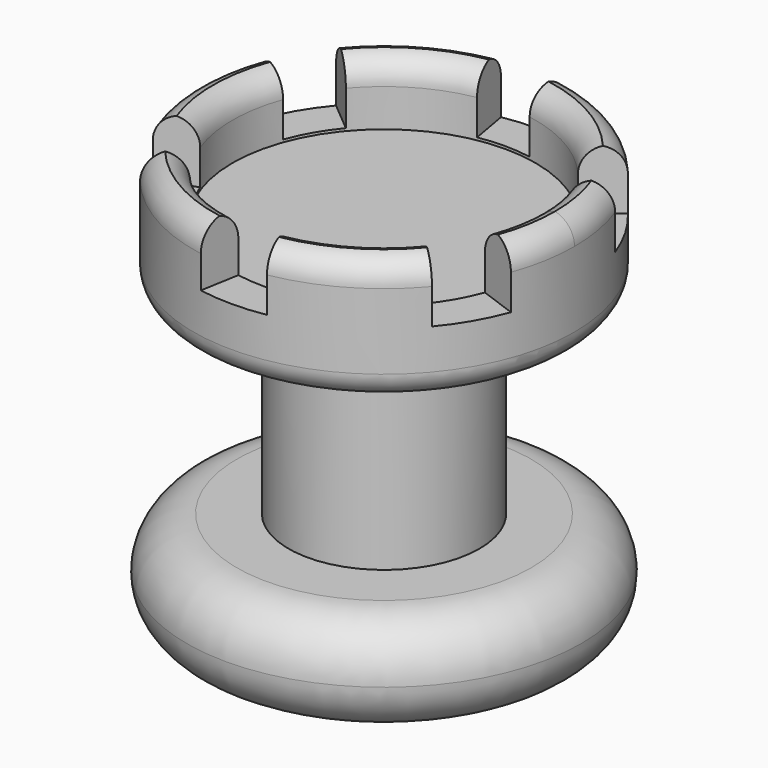
from build123d import *

# Parameters (mm, degrees)
F2_R          = 30.151436764
F3_DEPTH      = 12.5
F5_DEPTH      = 12
F6_R          = 9.99999
F7_T2_ANGLE   = 40
F7_T4_ANGLE   = 40
F8_T2_ANGLE   = 56.7791956191
F8_T4_ANGLE   = 61.1048655433
F9_T2_ANGLE   = 40
F9_T4_ANGLE   = 40
F10_T3_ANGLE  = 20
F10_T6_ANGLE  = 20
F10_T9_ANGLE  = 20
F10_T12_ANGLE = 20
F11_T2_ANGLE  = 40
F11_T4_ANGLE  = 40
F12_T2_ANGLE  = 87.5104431526
F12_T4_ANGLE  = 77.7726651693
F13_R         = 5


# Not quite as in the source:
# - a fillet or chamfer that OpenCascade refuses, or shapes differently, is made with other operations: its cross-section is extruded or revolved along the edge and cut away or added
# - a fillet or chamfer is up to 0.001 mm smaller than in the source, because OpenCascade refuses the exact size


with BuildPart() as f1:
    # F0 (on Front) → F1 (revolve)
    with BuildSketch(Plane.XZ):
        Polygon((0, 20), (0, 0), (19, 0), (39.2987092885, 0), (39.2987092885, 20), (19, 20), (19, 59.1294809732), (37.9244651105, 59.1294809732), (37.9244651105, 84.1294809732), (0, 84.1294809732), (0, 59.1294809732), align=None)
    revolve(axis=Axis((0, 0, 29.5647404866), (0, 0, 1)))

    # F2 (on face) → F3 (cut, symmetric)
    with BuildSketch(Plane.XY.offset(84.1294809732)):
        Circle(F2_R)
    extrude(amount=F3_DEPTH, both=True, mode=Mode.SUBTRACT)

    # F4 (on face) → F5 (cut)
    with BuildSketch(Plane.XY.offset(84.1294809732)):
        with BuildLine():
            ThreePointArc((-4.2811336318, 24.2795153332), (0, 24.654065993), (4.2811336318, 24.2795153332))
            Line((4.2811336318, 24.2795153332), (8.0445966017, 45.6231744531))
            ThreePointArc((8.0445966017, 45.6231744531), (0, 46.3269854584), (-8.0445966017, 45.6231744531))
            Line((-8.0445966017, 45.6231744531), (-4.2811336318, 24.2795153332))
        make_face()
        with BuildLine():
            ThreePointArc((-23.167243886, 8.4321871845), (-21.3510474565, 12.3270329965), (-18.8861102542, 15.8473281487))
            Line((-18.8861102542, 15.8473281487), (-35.4885297769, 29.7784122468))
            ThreePointArc((-35.4885297769, 29.7784122468), (-40.1203462877, 23.1634927292), (-43.5331263785, 15.8447622063))
            Line((-43.5331263785, 15.8447622063), (-23.167243886, 8.4321871845))
        make_face()
        with BuildLine():
            ThreePointArc((-18.8861102542, -15.8473281487), (-21.3510474565, -12.3270329965), (-23.167243886, -8.4321871845))
            Line((-23.167243886, -8.4321871845), (-43.5331263785, -15.8447622063))
            ThreePointArc((-43.5331263785, -15.8447622063), (-40.1203462877, -23.1634927292), (-35.4885297769, -29.7784122468))
            Line((-35.4885297769, -29.7784122468), (-18.8861102542, -15.8473281487))
        make_face()
        with BuildLine():
            ThreePointArc((4.2811336318, -24.2795153332), (0, -24.654065993), (-4.2811336318, -24.2795153332))
            Line((-4.2811336318, -24.2795153332), (-8.0445966017, -45.6231744531))
            ThreePointArc((-8.0445966017, -45.6231744531), (0, -46.3269854584), (8.0445966017, -45.6231744531))
            Line((8.0445966017, -45.6231744531), (4.2811336318, -24.2795153332))
        make_face()
        with BuildLine():
            ThreePointArc((23.167243886, -8.4321871845), (21.3510474565, -12.3270329965), (18.8861102542, -15.8473281487))
            Line((18.8861102542, -15.8473281487), (35.4885297769, -29.7784122468))
            ThreePointArc((35.4885297769, -29.7784122468), (40.1203462877, -23.1634927292), (43.5331263785, -15.8447622063))
            Line((43.5331263785, -15.8447622063), (23.167243886, -8.4321871845))
        make_face()
        with BuildLine():
            ThreePointArc((18.8861102542, 15.8473281487), (21.3510474565, 12.3270329965), (23.167243886, 8.4321871845))
            Line((23.167243886, 8.4321871845), (43.5331263785, 15.8447622063))
            ThreePointArc((43.5331263785, 15.8447622063), (40.1203462877, 23.1634927292), (35.4885297769, 29.7784122468))
            Line((35.4885297769, 29.7784122468), (18.8861102542, 15.8473281487))
        make_face()
    extrude(amount=-F5_DEPTH, mode=Mode.SUBTRACT)

    # F6 (radius 10 in the source; OpenCascade refuses exactly that, so slightly less here)
    f6_edges = [f1.edges().sort_by_distance(p)[0] for p in [
        (-39.298709, 0, 20),
        (-39.298709, 0, 0),
    ]]
    fillet(f6_edges, radius=F6_R)

    # F7: fillet of radius 5 on 2 edges, made by hand

    # F7_s1 → F7_t2 (revolve, cut)
    with BuildSketch(Plane(origin=(0, 0, 0), x_dir=(0, 0, 1), z_dir=(-0.984807753, -0.1736481777, 0))):
        with BuildLine():
            ThreePointArc((79.1294809732, -37.9244651105), (82.6650148792, -36.4599990164), (84.1294809732, -32.9244651105))
            Line((84.1294809732, -32.9244651105), (84.2294809732, -32.9244651105))
            Line((84.2294809732, -32.9244651105), (84.2294809732, -38.0244651105))
            Line((84.2294809732, -38.0244651105), (79.1294809732, -38.0244651105))
            Line((79.1294809732, -38.0244651105), (79.1294809732, -37.9244651105))
        make_face()
    revolve(axis=Axis((0, 0, 84.1294809732), (0, 0, 1)), revolution_arc=F7_T2_ANGLE, mode=Mode.SUBTRACT)

    # F7_s3 → F7_t4 (revolve, cut)
    with BuildSketch(Plane(origin=(0, 0, 0), x_dir=(0, 0, 1), z_dir=(-0.984807753, -0.1736481777, 0))):
        with BuildLine():
            ThreePointArc((84.1294809732, -35.151436764), (82.6650148792, -31.615902858), (79.1294809732, -30.151436764))
            Line((79.1294809732, -30.151436764), (79.1294809732, -30.051436764))
            Line((79.1294809732, -30.051436764), (84.2294809732, -30.051436764))
            Line((84.2294809732, -30.051436764), (84.2294809732, -35.151436764))
            Line((84.2294809732, -35.151436764), (84.1294809732, -35.151436764))
        make_face()
    revolve(axis=Axis((0, 0, 84.1294809732), (0, 0, 1)), revolution_arc=F7_T4_ANGLE, mode=Mode.SUBTRACT)

    # F8: fillet of radius 5.5526911935 on 2 edges, made by hand

    # F8_s1 → F8_t2 (revolve, cut)
    with BuildSketch(Plane(origin=(0, 0, 0), x_dir=(0, 0, 1), z_dir=(-0.5241405305, 0.8516317892, 0))):
        with BuildLine():
            ThreePointArc((78.5767897798, -37.9244651105), (82.5031353765, -36.2981195138), (84.1294809732, -32.371773917))
            Line((84.1294809732, -32.371773917), (84.2405347971, -32.371773917))
            Line((84.2405347971, -32.371773917), (84.2405347971, -38.0355189344))
            Line((84.2405347971, -38.0355189344), (78.5767897798, -38.0355189344))
            Line((78.5767897798, -38.0355189344), (78.5767897798, -37.9244651105))
        make_face()
    revolve(axis=Axis((0, 0, 84.1294809732), (0, 0, 1)), revolution_arc=F8_T2_ANGLE, mode=Mode.SUBTRACT)

    # F8_s3 → F8_t4 (revolve, cut)
    with BuildSketch(Plane(origin=(0, 0, 0), x_dir=(0, 0, 1), z_dir=(-0.4916268702, 0.8708059603, 0))):
        with BuildLine():
            ThreePointArc((84.1294809732, -35.7041279574), (82.5031353765, -31.7777823607), (78.5767897798, -30.151436764))
            Line((78.5767897798, -30.151436764), (78.5767897798, -30.0403829401))
            Line((78.5767897798, -30.0403829401), (84.2405347971, -30.0403829401))
            Line((84.2405347971, -30.0403829401), (84.2405347971, -35.7041279574))
            Line((84.2405347971, -35.7041279574), (84.1294809732, -35.7041279574))
        make_face()
    revolve(axis=Axis((0, 0, 84.1294809732), (0, 0, 1)), revolution_arc=F8_T4_ANGLE, mode=Mode.SUBTRACT)

    # F9: fillet of radius 5 on 2 edges, made by hand

    # F9_s1 → F9_t2 (revolve, cut)
    with BuildSketch(Plane(origin=(0, 0, 0), x_dir=(0, 0, 1), z_dir=(0.3420201433, 0.9396926208, 0))):
        with BuildLine():
            ThreePointArc((84.1294809732, -35.151436764), (82.6650148792, -31.615902858), (79.1294809732, -30.151436764))
            Line((79.1294809732, -30.151436764), (79.1294809732, -30.051436764))
            Line((79.1294809732, -30.051436764), (84.2294809732, -30.051436764))
            Line((84.2294809732, -30.051436764), (84.2294809732, -35.151436764))
            Line((84.2294809732, -35.151436764), (84.1294809732, -35.151436764))
        make_face()
    revolve(axis=Axis((0, 0, 84.1294809732), (0, 0, 1)), revolution_arc=F9_T2_ANGLE, mode=Mode.SUBTRACT)

    # F9_s3 → F9_t4 (revolve, cut)
    with BuildSketch(Plane(origin=(0, 0, 0), x_dir=(0, 0, 1), z_dir=(0.3420201433, 0.9396926208, 0))):
        with BuildLine():
            ThreePointArc((79.1294809732, -37.9244651105), (82.6650148792, -36.4599990164), (84.1294809732, -32.9244651105))
            Line((84.1294809732, -32.9244651105), (84.2294809732, -32.9244651105))
            Line((84.2294809732, -32.9244651105), (84.2294809732, -38.0244651105))
            Line((84.2294809732, -38.0244651105), (79.1294809732, -38.0244651105))
            Line((79.1294809732, -38.0244651105), (79.1294809732, -37.9244651105))
        make_face()
    revolve(axis=Axis((0, 0, 84.1294809732), (0, 0, 1)), revolution_arc=F9_T4_ANGLE, mode=Mode.SUBTRACT)

    # F10: fillet of radius 5 on 2 edges, made by hand


with BuildPart() as f10_tool1:
    # F10_s2 → F10_t3 (revolve)
    with BuildSketch(Plane(origin=(0, 0, 0), x_dir=(0, 0, 1), z_dir=(-0.3420201433, -0.9396926208, 0))):
        with BuildLine():
            ThreePointArc((84.1294809732, -35.151436764), (82.6650148792, -31.615902858), (79.1294809732, -30.151436764))
            Line((79.1294809732, -30.151436764), (79.1294809732, -30.051436764))
            Line((79.1294809732, -30.051436764), (84.2294809732, -30.051436764))
            Line((84.2294809732, -30.051436764), (84.2294809732, -35.151436764))
            Line((84.2294809732, -35.151436764), (84.1294809732, -35.151436764))
        make_face()
    revolve(axis=Axis((0, 0, 84.1294809732), (0, 0, 1)), revolution_arc=F10_T3_ANGLE)


with BuildPart() as f10_tool4:
    # F10_s5 → F10_t6 (revolve)
    with BuildSketch(Plane(origin=(0, 0, 0), x_dir=(0, 0, 1), z_dir=(-0.3420201433, -0.9396926208, 0))):
        with BuildLine():
            ThreePointArc((79.1294809732, -37.9244651105), (82.6650148792, -36.4599990164), (84.1294809732, -32.9244651105))
            Line((84.1294809732, -32.9244651105), (84.2294809732, -32.9244651105))
            Line((84.2294809732, -32.9244651105), (84.2294809732, -38.0244651105))
            Line((84.2294809732, -38.0244651105), (79.1294809732, -38.0244651105))
            Line((79.1294809732, -38.0244651105), (79.1294809732, -37.9244651105))
        make_face()
    revolve(axis=Axis((0, 0, 84.1294809732), (0, 0, 1)), revolution_arc=F10_T6_ANGLE)


with BuildPart() as f10_tool7:
    # F10_s8 → F10_t9 (revolve)
    with BuildSketch(Plane.XZ):
        with BuildLine():
            ThreePointArc((37.9244651105, 79.1294809732), (36.4599990164, 82.6650148792), (32.9244651105, 84.1294809732))
            Line((32.9244651105, 84.1294809732), (32.9244651105, 84.2294809732))
            Line((32.9244651105, 84.2294809732), (38.0244651105, 84.2294809732))
            Line((38.0244651105, 84.2294809732), (38.0244651105, 79.1294809732))
            Line((38.0244651105, 79.1294809732), (37.9244651105, 79.1294809732))
        make_face()
    revolve(axis=Axis((0, 0, 84.1294809732), (0, 0, 1)), revolution_arc=F10_T9_ANGLE)


with BuildPart() as f10_tool10:
    # F10_s11 → F10_t12 (revolve)
    with BuildSketch(Plane.XZ):
        with BuildLine():
            ThreePointArc((35.151436764, 84.1294809732), (31.615902858, 82.6650148792), (30.151436764, 79.1294809732))
            Line((30.151436764, 79.1294809732), (30.051436764, 79.1294809732))
            Line((30.051436764, 79.1294809732), (30.051436764, 84.2294809732))
            Line((30.051436764, 84.2294809732), (35.151436764, 84.2294809732))
            Line((35.151436764, 84.2294809732), (35.151436764, 84.1294809732))
        make_face()
    revolve(axis=Axis((0, 0, 84.1294809732), (0, 0, 1)), revolution_arc=F10_T12_ANGLE)


with BuildPart() as f1_1:
    add(f1.part)

    # F10_t13: cut F10_tool1, F10_tool4, F10_tool7, F10_tool10
    add([f10_tool1.part, f10_tool4.part, f10_tool7.part, f10_tool10.part], mode=Mode.SUBTRACT)

    # F11: fillet of radius 5 on 2 edges, made by hand

    # F11_s1 → F11_t2 (revolve, cut)
    with BuildSketch(Plane(origin=(0, 0, 0), x_dir=(0, 0, 1), z_dir=(0.6427876097, -0.7660444431, 0))):
        with BuildLine():
            ThreePointArc((79.1294809732, -30.151436764), (82.6650148792, -31.615902858), (84.1294809732, -35.151436764))
            Line((84.1294809732, -35.151436764), (84.2294809732, -35.151436764))
            Line((84.2294809732, -35.151436764), (84.2294809732, -30.051436764))
            Line((84.2294809732, -30.051436764), (79.1294809732, -30.051436764))
            Line((79.1294809732, -30.051436764), (79.1294809732, -30.151436764))
        make_face()
    revolve(axis=Axis((0, 0, 84.1294809732), (0, 0, 1)), revolution_arc=F11_T2_ANGLE, mode=Mode.SUBTRACT)

    # F11_s3 → F11_t4 (revolve, cut)
    with BuildSketch(Plane(origin=(0, 0, 0), x_dir=(0, 0, 1), z_dir=(0.6427876097, -0.7660444431, 0))):
        with BuildLine():
            ThreePointArc((79.1294809732, -37.9244651105), (82.6650148792, -36.4599990164), (84.1294809732, -32.9244651105))
            Line((84.1294809732, -32.9244651105), (84.2294809732, -32.9244651105))
            Line((84.2294809732, -32.9244651105), (84.2294809732, -38.0244651105))
            Line((84.2294809732, -38.0244651105), (79.1294809732, -38.0244651105))
            Line((79.1294809732, -38.0244651105), (79.1294809732, -37.9244651105))
        make_face()
    revolve(axis=Axis((0, 0, 84.1294809732), (0, 0, 1)), revolution_arc=F11_T4_ANGLE, mode=Mode.SUBTRACT)

    # F12: fillet of radius 5 on 2 edges, made by hand

    # F12_s1 → F12_t2 (revolve, cut)
    with BuildSketch(Plane(origin=(0, 0, 0), x_dir=(0, 0, 1), z_dir=(0.9713204046, -0.2377744133, 0))):
        with BuildLine():
            ThreePointArc((84.1294809732, -35.151436764), (82.6650148792, -31.615902858), (79.1294809732, -30.151436764))
            Line((79.1294809732, -30.151436764), (84.1294809732, -30.151436764))
            Line((84.1294809732, -30.151436764), (84.1294809732, -35.151436764))
        make_face()
    revolve(axis=Axis((0, 0, 84.1294809732), (0, 0, 1)), revolution_arc=F12_T2_ANGLE, mode=Mode.SUBTRACT)

    # F12_s3 → F12_t4 (revolve, cut)
    with BuildSketch(Plane(origin=(0, 0, 0), x_dir=(0, 0, 1), z_dir=(0.9879967425, -0.1544747126, 0))):
        with BuildLine():
            ThreePointArc((79.1294809732, -37.9244651105), (82.6650148792, -36.4599990164), (84.1294809732, -32.9244651105))
            Line((84.1294809732, -32.9244651105), (84.1294809732, -37.9244651105))
            Line((84.1294809732, -37.9244651105), (79.1294809732, -37.9244651105))
        make_face()
    revolve(axis=Axis((0, 0, 84.1294809732), (0, 0, 1)), revolution_arc=F12_T4_ANGLE, mode=Mode.SUBTRACT)

    # F13
    f13_edges = [f1_1.edges().sort_by_distance(p)[0] for p in [
        (-37.924465, 0, 59.129481),
        (-19, 0, 59.129481),
    ]]
    fillet(f13_edges, radius=F13_R)


solid = f1_1.part
